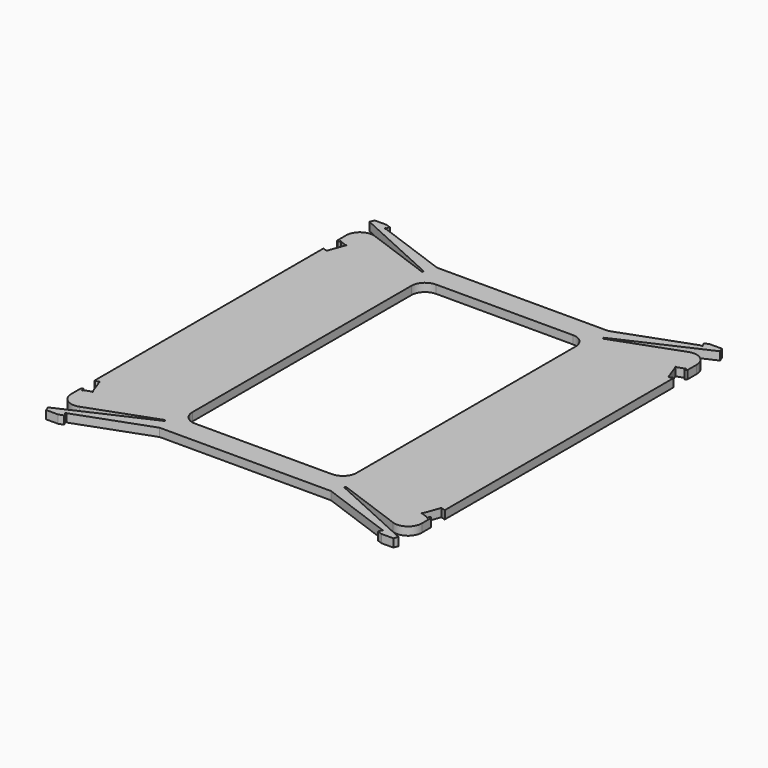
from build123d import *

# Parameters (mm, degrees)
F1_DEPTH = 1.5
F4_W     = 60
F4_H     = 110
F5_DEPTH = 3
F6_R     = 5
F7_R     = 5


# Not quite as in the source:
# - a feature names something its author has since deleted; it is built from what else it names


with BuildPart() as f1:
    # F0 (on Top) → F1 (new body, symmetric)
    with BuildSketch(Plane.XY):
        with BuildLine():
            Line((31.2800427974, 63.3035998776), (0, 63.3035998776))
            Line((0, 63.3035998776), (0, 0))
            Line((0, 0), (64, 0))
            Line((64, 0), (64, 52.0472386562))
            ThreePointArc((64, 52.0472386562), (63.9147152873, 52.211069065), (63.7315959713, 52.2351771803))
            Line((63.7315959713, 52.2351771803), (62.4040530693, 51.7519910793))
            Line((62.4040530693, 51.7519910793), (60.2493261663, 57.6720545902))
            ThreePointArc((60.2493261663, 57.6720545902), (59.9996605802, 57.9445167667), (60.3688606618, 57.9283971431))
            Line((60.3688606618, 57.9283971431), (62.8120614758, 58.8176495157))
            ThreePointArc((62.8120614758, 58.8176495157), (63.0845236523, 59.0673151018), (63.0684040287, 58.6981150202))
            Line((63.0684040287, 58.6981150202), (63.2443290661, 58.2147649522))
            ThreePointArc((63.2443290661, 58.2147649522), (63.3805037813, 58.0899838157), (63.5608251122, 58.1299600923))
            Line((63.5608251122, 58.1299600923), (63.9285575219, 58.4385242216))
            ThreePointArc((63.9285575219, 58.4385242216), (63.9812615574, 58.5072094579), (64, 58.5917331103))
            Line((64, 58.5917331103), (64, 69.8918015034))
            Line((64, 69.8918015034), (32.9901435141, 58.6051367736))
            Line((32.9901435141, 58.6051367736), (32.7849314281, 59.1689523461))
            Line((32.7849314281, 59.1689523461), (64, 73.3944786626))
            Line((64, 73.3944786626), (63.4156380227, 75))
            Line((63.4156380227, 75), (59.0299314225, 75))
            Line((59.0299314225, 75), (57.3566676351, 74.3909817873))
            Line((57.3566676351, 74.3909817873), (57.8012938214, 73.1693813803))
            ThreePointArc((57.8012938214, 73.1693813803), (58.0509594075, 72.8969192038), (57.681759326, 72.9130388275))
            Line((57.681759326, 72.9130388275), (31.2800427974, 63.3035998776))
        make_face()
    extrude(amount=F1_DEPTH, both=True)

    # F2: F1 across face


with BuildPart() as f1_1:
    add(f1.part)
    add(f1.part.mirror(Plane(origin=(0, 31.6517999388, 0), x_dir=(0, -1, 0), z_dir=(-1, 0, 0))))

    # F3: F1 across face


with BuildPart() as f1_2:
    add(f1_1.part)
    add(f1_1.part.mirror(Plane.XZ))

    # F4 (on face) → F5 (cut, through all)
    with BuildSketch(Plane(origin=(0, 0, -1.5), x_dir=(1, 0, 0), z_dir=(0, 0, -1))):
        Rectangle(F4_W, F4_H)
    extrude(amount=-F5_DEPTH, mode=Mode.SUBTRACT)

    # F6
    f6_edges = [f1_2.edges().sort_by_distance(p)[0] for p in [
        (-64, -69.891802, 0),
        (64, -69.891802, 0),
        (64, 69.891802, 0),
        (-64, 69.891802, 0),
    ]]
    fillet(f6_edges, radius=F6_R)

    # F7
    f7_edges = [f1_2.edges().sort_by_distance(p)[0] for p in [
        (-30, 55, 0),
        (-30, -55, 0),
        (30, -55, 0),
        (30, 55, 0),
    ]]
    fillet(f7_edges, radius=F7_R)


solid = f1_2.part
